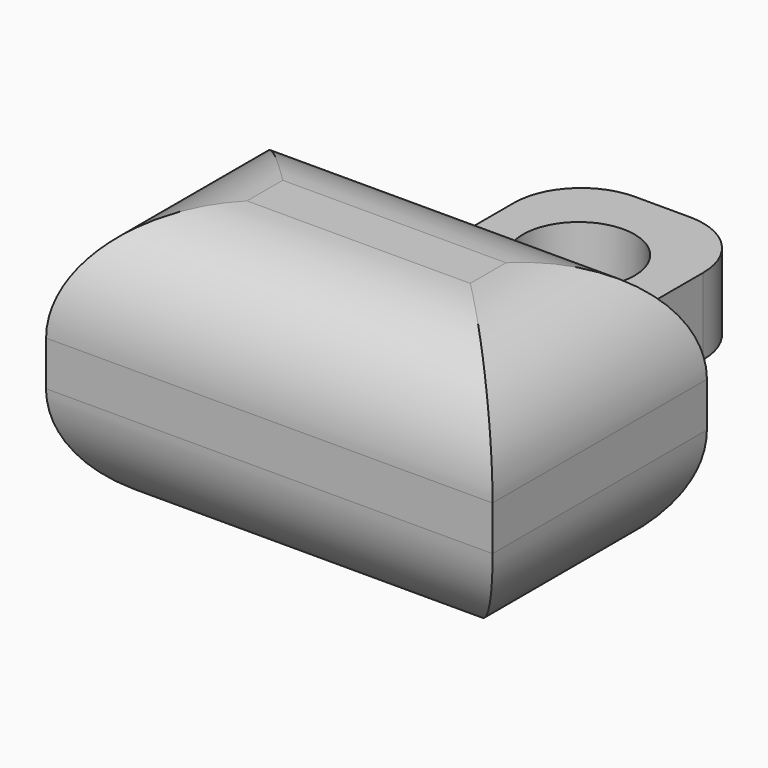
from build123d import *

# Parameters (mm, degrees)
F0_W         = 100
F0_H         = 60
F1_DEPTH     = 60
F2_W         = 42.3733331263
F2_H         = 17.1486828476
F3_DEPTH     = 50
F4_R         = 12.5
F5_DEPTH     = 32.4145003611
F6_T1_DEPTH  = 185
F6_T3_DEPTH  = 225
F6_T8_DEPTH  = 225
F6_T14_DEPTH = 225
F6_T20_DEPTH = 225
F6_T27_DEPTH = 225
F6_T33_DEPTH = 225
F7_R         = 15


# Not quite as in the source:
# - a fillet or chamfer that OpenCascade refuses, or shapes differently, is made with other operations: its cross-section is extruded or revolved along the edge and cut away or added


with BuildPart() as f1:
    # F0 (on Top) → F1 (new body)
    with BuildSketch(Plane.XY):
        Rectangle(F0_W, F0_H)
    extrude(amount=F1_DEPTH)

    # F2 (on face) → F3 (join)
    with BuildSketch(Plane(origin=(0, 30, 0), x_dir=(-1, 0, 0), z_dir=(0, 1, 0))):
        with Locations((0, 23.8391589373)):
            Rectangle(F2_W, F2_H)
    extrude(amount=F3_DEPTH)

    # F4 (on face) → F5 (cut, through all)
    with BuildSketch(Plane.XY.offset(32.4135003611)):
        with Locations((0, 56.6370971501)):
            Circle(F4_R)
    extrude(amount=-F5_DEPTH, mode=Mode.SUBTRACT)

    # F6: fillet of radius 25 on 8 edges, made by hand

    # F6_s2 → F6_t1 (cut)
    with BuildSketch(Plane.XZ.offset(-92.5)):
        with BuildLine():
            ThreePointArc((-50, 35), (-42.6776695297, 52.6776695297), (-25, 60))
            Line((-25, 60), (-50, 60))
            Line((-50, 60), (-50, 35))
        make_face()
        with BuildLine():
            ThreePointArc((25, 60), (42.6776695297, 52.6776695297), (50, 35))
            Line((50, 35), (50, 60))
            Line((50, 60), (25, 60))
        make_face()
        with BuildLine():
            ThreePointArc((-50, 25), (-42.6776695297, 7.3223304703), (-25, 0))
            Line((-25, 0), (-50, 0))
            Line((-50, 0), (-50, 25))
        make_face()
        with BuildLine():
            ThreePointArc((25, 0), (42.6776695297, 7.3223304703), (50, 25))
            Line((50, 25), (50, 0))
            Line((50, 0), (25, 0))
        make_face()
    extrude(amount=F6_T1_DEPTH, mode=Mode.SUBTRACT)

    # F6_s4 → F6_t3 (cut)
    with BuildSketch(Plane.YZ.offset(-112.5)):
        with BuildLine():
            ThreePointArc((-30, 35), (-22.6776695297, 52.6776695297), (-5, 60))
            Line((-5, 60), (-30, 60))
            Line((-30, 60), (-30, 35))
        make_face()
        with BuildLine():
            ThreePointArc((30, 35), (22.6776695297, 52.6776695297), (5, 60))
            Line((5, 60), (30, 60))
            Line((30, 60), (30, 35))
        make_face()
        with BuildLine():
            ThreePointArc((-30, 25), (-22.6776695297, 7.3223304703), (-5, 0))
            Line((-5, 0), (-30, 0))
            Line((-30, 0), (-30, 25))
        make_face()
    extrude(amount=F6_T3_DEPTH, mode=Mode.SUBTRACT)


with BuildPart() as f6_tool6:
    # F6_s7 → F6_t8 (new body)
    with BuildSketch(Plane.YZ.offset(112.5)):
        with BuildLine():
            ThreePointArc((30, 25), (22.6776695297, 7.3223304703), (5, 0))
            Line((5, 0), (30, 0))
            Line((30, 0), (30, 25))
        make_face()
    extrude(amount=-F6_T8_DEPTH)

    split(bisect_by=Plane.XY.offset(15.2648175135), keep=Keep.TOP)

    split(bisect_by=Plane.YZ.offset(21.1866665632), keep=Keep.TOP)


with BuildPart() as f1_1:
    add(f1.part)

    # F6_t5: cut F6_tool6
    add(f6_tool6.part, mode=Mode.SUBTRACT)


with BuildPart() as f6_tool12:
    # F6_s13 → F6_t14 (new body)
    with BuildSketch(Plane.YZ.offset(112.5)):
        with BuildLine():
            ThreePointArc((30, 25), (22.6776695297, 7.3223304703), (5, 0))
            Line((5, 0), (30, 0))
            Line((30, 0), (30, 25))
        make_face()
    extrude(amount=-F6_T14_DEPTH)

    split(bisect_by=Plane.XY.offset(15.2648175135), keep=Keep.BOTTOM)

    split(bisect_by=Plane.YZ.offset(21.1866665632), keep=Keep.TOP)


with BuildPart() as f1_2:
    add(f1_1.part)

    # F6_t11: cut F6_tool12
    add(f6_tool12.part, mode=Mode.SUBTRACT)


with BuildPart() as f6_tool18:
    # F6_s19 → F6_t20 (new body)
    with BuildSketch(Plane.YZ.offset(112.5)):
        with BuildLine():
            ThreePointArc((30, 25), (22.6776695297, 7.3223304703), (5, 0))
            Line((5, 0), (30, 0))
            Line((30, 0), (30, 25))
        make_face()
    extrude(amount=-F6_T20_DEPTH)

    split(bisect_by=Plane.XY.offset(15.2648175135), keep=Keep.BOTTOM)

    split(bisect_by=Plane.YZ.offset(21.1866665632), keep=Keep.BOTTOM)

    split(bisect_by=Plane.YZ.offset(-21.1866665632), keep=Keep.TOP)


with BuildPart() as f1_3:
    add(f1_2.part)

    # F6_t17: cut F6_tool18
    add(f6_tool18.part, mode=Mode.SUBTRACT)


with BuildPart() as f6_tool25:
    # F6_s26 → F6_t27 (new body)
    with BuildSketch(Plane.YZ.offset(112.5)):
        with BuildLine():
            ThreePointArc((30, 25), (22.6776695297, 7.3223304703), (5, 0))
            Line((5, 0), (30, 0))
            Line((30, 0), (30, 25))
        make_face()
    extrude(amount=-F6_T27_DEPTH)

    split(bisect_by=Plane.XY.offset(15.2648175135), keep=Keep.TOP)

    split(bisect_by=Plane.YZ.offset(-21.1866665632), keep=Keep.BOTTOM)


with BuildPart() as f1_4:
    add(f1_3.part)

    # F6_t24: cut F6_tool25
    add(f6_tool25.part, mode=Mode.SUBTRACT)


with BuildPart() as f6_tool31:
    # F6_s32 → F6_t33 (new body)
    with BuildSketch(Plane.YZ.offset(112.5)):
        with BuildLine():
            ThreePointArc((30, 25), (22.6776695297, 7.3223304703), (5, 0))
            Line((5, 0), (30, 0))
            Line((30, 0), (30, 25))
        make_face()
    extrude(amount=-F6_T33_DEPTH)

    split(bisect_by=Plane.XY.offset(15.2648175135), keep=Keep.BOTTOM)

    split(bisect_by=Plane.YZ.offset(-21.1866665632), keep=Keep.BOTTOM)


with BuildPart() as f1_5:
    add(f1_4.part)

    # F6_t30: cut F6_tool31
    add(f6_tool31.part, mode=Mode.SUBTRACT)

    # F7
    f7_edges = [f1_5.edges().sort_by_distance(p)[0] for p in [
        (-21.186667, 80, 23.839159),
        (21.186667, 80, 23.839159),
    ]]
    fillet(f7_edges, radius=F7_R)


solid = f1_5.part
